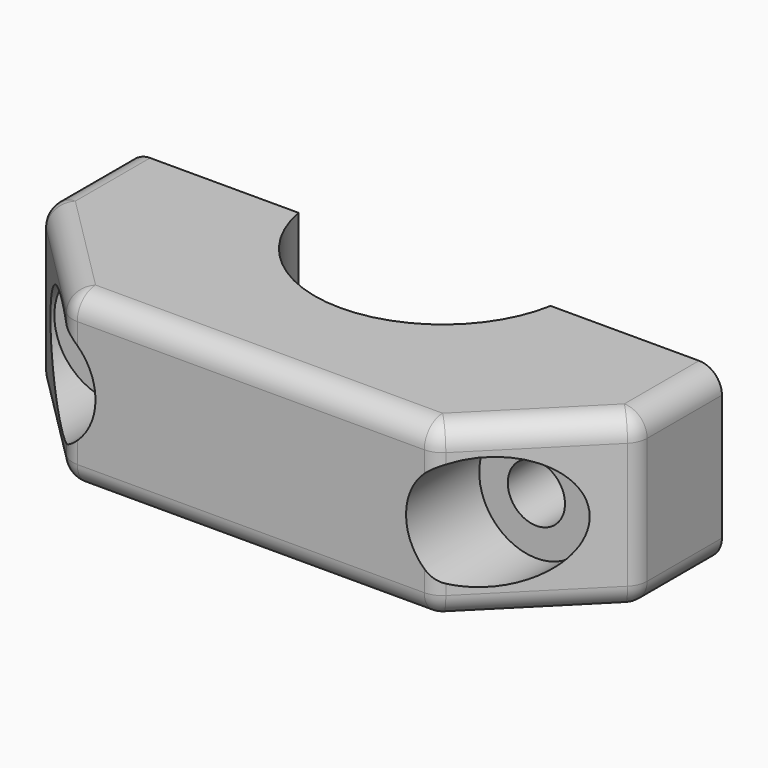
from build123d import *

# Parameters (mm, degrees)
F1_DEPTH       = 15
F2_DEPTH       = 5
F3_DEPTH       = 5
F5_D           = 5
F5_CBORE_D     = 10
F5_CBORE_DEPTH = 8
F6_T1_DEPTH    = 66.4336597593
F7_R           = 2
F8_W           = 54.7069119513
F8_H           = 16.1263942719
F9_DEPTH       = 1


# Not quite as in the source:
# - a fillet or chamfer that OpenCascade refuses, or shapes differently, is made with other operations: its cross-section is extruded or revolved along the edge and cut away or added


with BuildPart() as f1:
    # F0 (on Top) → F1 (new body)
    with BuildSketch(Plane.XY):
        with BuildLine():
            Line((-21, -10), (21, -10))
            Line((21, -10), (21, 10))
            Line((21, 10), (11.1552678139, 10))
            ThreePointArc((11.1552678139, 10), (0, -0.2), (-11.1552678139, 10))
            Line((-11.1552678139, 10), (-21, 10))
            Line((-21, 10), (-21, -10))
        make_face()
    extrude(amount=F1_DEPTH)

    # F2 (add): a face of the model
    f2_faces = [f1.faces().sort_by_distance(p)[0] for p in [
        (21, 0, 7.5),
    ]]
    extrude(f2_faces, amount=F2_DEPTH)

    # F3 (add): a face of the model
    f3_faces = [f1.faces().sort_by_distance(p)[0] for p in [
        (-21, 0, 7.5),
    ]]
    extrude(f3_faces, amount=F3_DEPTH)

    # F5 (through all)
    with Locations(Plane.XZ.offset(10)):
        with Locations((18.577633907, 7.5), (-18.577633907, 7.5)):
            CounterBoreHole(F5_D / 2, F5_CBORE_D / 2, F5_CBORE_DEPTH)

    # F6: chamfer of 10 on 2 edges, made by hand

    # F6_s2 → F6_t1 (cut)
    with BuildSketch(Plane.XY.offset(-25.7168298797)):
        Polygon((16, -10), (26, 0), (26, -10), align=None)
        Polygon((-26, 0), (-16, -10), (-26, -10), align=None)
    extrude(amount=F6_T1_DEPTH, mode=Mode.SUBTRACT)

    # F7
    f7_edges = [f1.edges().sort_by_distance(p)[0] for p in [
        (0, -10, 15),
        (21, -5, 15),
        (-26, 5, 15),
        (26, 5, 15),
        (-21, -5, 15),
        (21, -5, 0),
        (0, -10, 0),
        (-21, -5, 0),
        (26, 5, 0),
        (-26, 5, 0),
        (16, -10, 13.392184),
        (16, -10, 1.607816),
        (-16, -10, 1.607816),
        (-16, -10, 13.392184),
        (26, 0, 7.5),
        (-26, 0, 7.5),
    ]]
    fillet(f7_edges, radius=F7_R)

    # F8 (on face) → F9 (cut)
    with BuildSketch(Plane(origin=(0, 10, 0), x_dir=(-1, 0, 0), z_dir=(0, 1, 0))):
        with Locations((-1.3534559757, 8.0631971359)):
            Rectangle(F8_W, F8_H)
    extrude(amount=-F9_DEPTH, mode=Mode.SUBTRACT)


solid = f1.part
